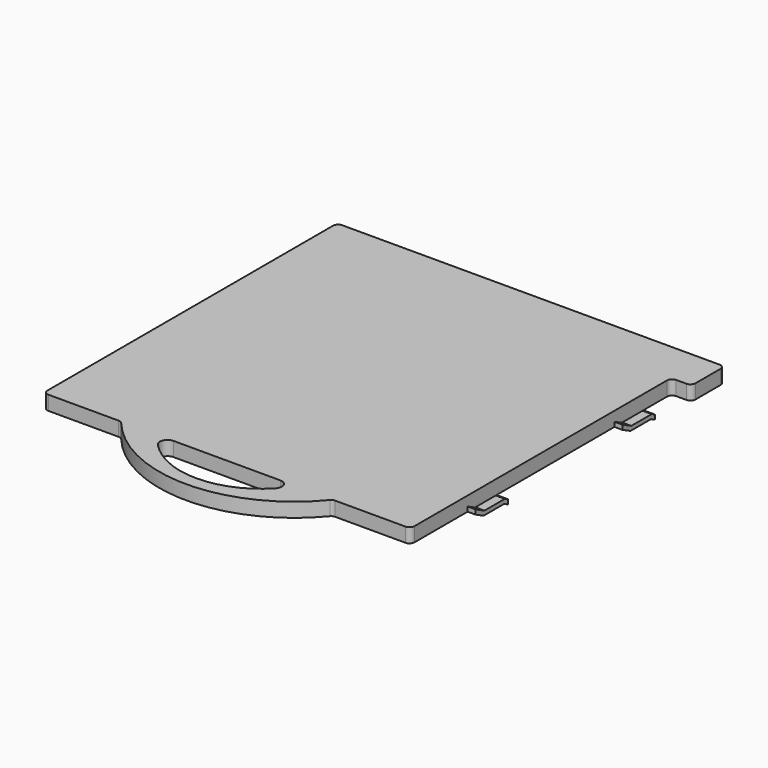
from build123d import *

# Parameters (mm, degrees)
F1_DEPTH      = 8.89
F3_DEPTH      = 4.9276
F3_DEPTH_BACK = 2.54
F7_DEPTH      = 13.6535


with BuildPart() as f1:
    # F0 (on Top) → F1 (new body)
    with BuildSketch(Plane.XY):
        with BuildLine():
            Line((67.3940027121, -114.3), (111.125, -114.3))
            ThreePointArc((111.125, -114.3), (113.3700640303, -113.3700640303), (114.3, -111.125))
            Line((114.3, -111.125), (114.3, 85.344))
            ThreePointArc((114.3, 85.344), (115.2299359697, 87.5890640303), (117.475, 88.519))
            Line((117.475, 88.519), (123.825, 88.519))
            ThreePointArc((123.825, 88.519), (126.0700640303, 89.4489359697), (127, 91.694))
            Line((127, 91.694), (127, 111.125))
            ThreePointArc((127, 111.125), (126.0700640303, 113.3700640303), (123.825, 114.3))
            Line((123.825, 114.3), (114.3, 114.3))
            Line((114.3, 114.3), (-111.125, 114.3))
            ThreePointArc((-111.125, 114.3), (-113.3700640303, 113.3700640303), (-114.3, 111.125))
            Line((-114.3, 111.125), (-114.3, -111.125))
            ThreePointArc((-114.3, -111.125), (-113.3700640303, -113.3700640303), (-111.125, -114.3))
            Line((-111.125, -114.3), (-67.3940027121, -114.3))
            ThreePointArc((-67.3940027121, -114.3), (-66.0408699293, -114.6027784431), (-64.9458155322, -115.4533658758))
            ThreePointArc((-64.9458155322, -115.4533658758), (0, -146.05), (64.9458155322, -115.4533658758))
            ThreePointArc((64.9458155322, -115.4533658758), (66.0408699293, -114.6027784431), (67.3940027121, -114.3))
        make_face()
    extrude(amount=F1_DEPTH)



with BuildPart() as f3:
    # F2 (on face) → F3 (new body, two sides)
    with BuildSketch(Plane.YZ.offset(114.3)) as f3_sk:
        Polygon((50.8, -3.175), (66.675, -3.175), (69.85, -4.7625), (69.85, -1.9226936686), (67.2746126628, -0.635), (51.3996126628, -0.635), (50.1296126628, 0), (44.45, 0), align=None)
        Polygon((44.45, 2.8398063314), (44.45, 0), (50.1296126628, 0), align=None)
    extrude(amount=F3_DEPTH)
    extrude(f3_sk.sketch, amount=-F3_DEPTH_BACK)


with BuildPart() as f4_1:
    # F4: copy of F3
    add(f3.part.moved(Location((0, -114.3, 0))))


with BuildPart() as f1_1:
    add(f1.part)

    add(f3.part)  # F5 merges F3

    add(f4_1.part)  # F5 merges F4_1
    # F5: F3, F4_1 across plane
    add(f3.part.mirror(Plane.YZ))
    add(f4_1.part.mirror(Plane.YZ))

    # F6 (on face) → F7 (cut, through all)
    with BuildSketch(Plane.XY.offset(8.89)):
        with BuildLine():
            Line((33.2011497354, -114.3), (-33.2011497354, -114.3))
            ThreePointArc((-33.2011497354, -114.3), (-37.5757853229, -117.1799565804), (-36.6596028328, -122.33671875))
            ThreePointArc((-36.6596028328, -122.33671875), (0, -138.1125), (36.6596028328, -122.33671875))
            ThreePointArc((36.6596028328, -122.33671875), (37.5757853229, -117.1799565804), (33.2011497354, -114.3))
        make_face()
    extrude(amount=-F7_DEPTH, mode=Mode.SUBTRACT)


solid = f1_1.part
